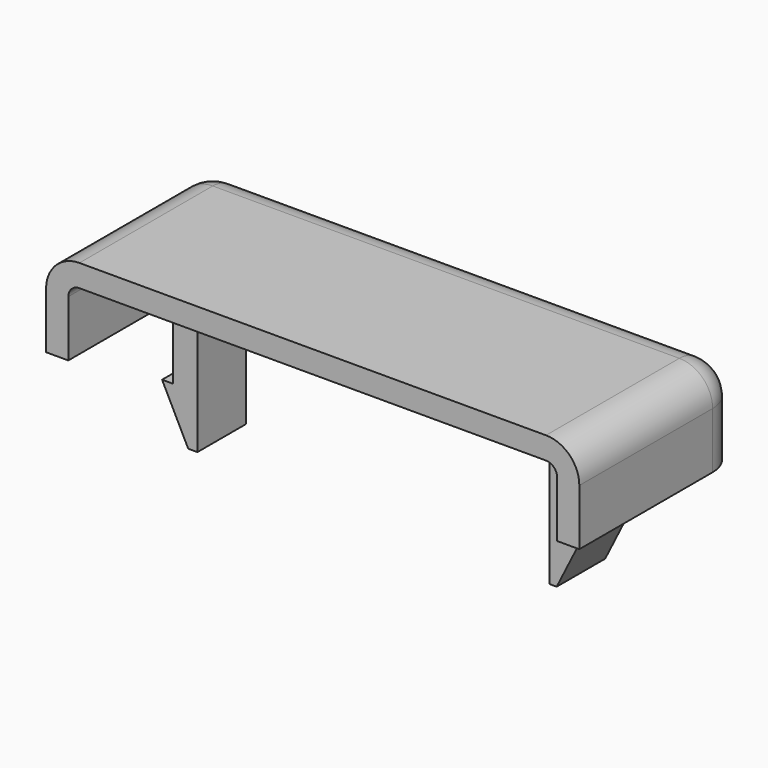
from build123d import *

# Parameters (mm, degrees)
F0_W         = 48
F0_H         = 8.0539090559
F1_DEPTH     = 18
F2_R         = 3
F3_T         = -2
F4_W         = 3.6368723959
F4_H         = 5.4553076625
F5_DEPTH     = 8
F6_W         = 3.8294224069
F6_H         = 5.4512945935
F7_DEPTH     = 8
F8_W         = 2.2997260094
F8_H         = 6.8176840032
F9_DEPTH     = 13.4
F8_W_2       = 2.9408568516
F11_T1_DEPTH = 36.529241079
F12_T1_DEPTH = 36.5332541479
F13_T1_DEPTH = 5.4512945935
F13_T3_DEPTH = 5.4553076625
F14_SIZE     = 1


# Not quite as in the source:
# - a fillet or chamfer that OpenCascade refuses, or shapes differently, is made with other operations: its cross-section is extruded or revolved along the edge and cut away or added


with BuildPart() as f1:
    # F0 (on Front) → F1 (new body)
    with BuildSketch(Plane.XZ):
        with Locations((7.3680209219, 4.0269545279)):
            Rectangle(F0_W, F0_H)
    extrude(amount=-F1_DEPTH)

    # F2
    f2_edges = [f1.edges().sort_by_distance(p)[0] for p in [
        (7.368021, 18, 8.053909),
        (-16.631979, 9, 8.053909),
        (31.368021, 9, 8.053909),
        (-16.631979, 18, 4.026955),
        (31.368021, 18, 4.026955),
    ]]
    fillet(f2_edges, radius=F2_R)

    # F3
    f3_openings = [f1.faces().sort_by_distance(p)[0] for p in [
        (7.368021, 0, 3.993074),
        (7.368021, 8.962591, 0),
    ]]
    offset(amount=F3_T, openings=f3_openings)

    # F4 (on Top) → F5 (join, symmetric)
    with BuildSketch(Plane.XY):
        with Locations((25.2722883597, 9.2779155821)):
            Rectangle(F4_W, F4_H)
    extrude(amount=F5_DEPTH, both=True)

    # F6 (on Top) → F7 (join, symmetric)
    with BuildSketch(Plane.XY):
        with Locations((-10.3424843401, 9.4998679124)):
            Rectangle(F6_W, F6_H)
    extrude(amount=F7_DEPTH, both=True)


with BuildPart() as f9:
    # F8 (on Front) → F9 (new body)
    with BuildSketch(Plane.XZ):
        with Locations((26.7013879493, 0.1128966487)):
            Rectangle(F8_W, F8_H)
    extrude(amount=-F9_DEPTH)


with BuildPart() as f9b:
    # F8 (on Front) → F9, piece 2 (new body)
    with BuildSketch(Plane.XZ):
        with Locations((-12.0930257253, 0.1128966487)):
            Rectangle(F8_W_2, F8_H)
    extrude(amount=-F9_DEPTH)


with BuildPart() as f1_1:
    add(f1.part)

    # F10: cut F9, F9b
    add(f9.part, mode=Mode.SUBTRACT)
    add(f9b.part, mode=Mode.SUBTRACT)

    # F11: chamfer of 6 x 3 on 1 edges, made by hand

    # F11_s2 → F11_t1 (cut)
    with BuildSketch(Plane.XZ.offset(-27.7644884519)):
        Polygon((-12.2571955435, -2), (-9.2571955435, -8), (-12.2571955435, -8), align=None)
    extrude(amount=F11_T1_DEPTH, mode=Mode.SUBTRACT)

    # F12: chamfer of 3 x 6 on 1 edges, made by hand

    # F12_s2 → F12_t1 (cut)
    with BuildSketch(Plane.XZ.offset(-27.544542656)):
        Polygon((27.0907245576, -2), (24.0907245576, -8), (27.0907245576, -8), align=None)
    extrude(amount=F12_T1_DEPTH, mode=Mode.SUBTRACT)

    # F13: fillet of radius 2 on 4 edges, made by hand

    # F13_s2 → F13_t1 (join)
    with BuildSketch(Plane.XZ.offset(-12.2255152091)):
        with BuildLine():
            ThreePointArc((-6.4277731366, 6.0539090559), (-7.841986699, 5.4681226183), (-8.4277731366, 4.0539090559))
            Line((-8.4277731366, 4.0539090559), (-8.4677731366, 4.0539090559))
            Line((-8.4677731366, 4.0539090559), (-8.4677731366, 6.0939090559))
            Line((-8.4677731366, 6.0939090559), (-6.4277731366, 6.0939090559))
            Line((-6.4277731366, 6.0939090559), (-6.4277731366, 6.0539090559))
        make_face()
        with BuildLine():
            ThreePointArc((-14.2571955435, 6.0539090559), (-12.8429819811, 5.4681226183), (-12.2571955435, 4.0539090559))
            Line((-12.2571955435, 4.0539090559), (-12.2171955435, 4.0539090559))
            Line((-12.2171955435, 4.0539090559), (-12.2171955435, 6.0939090559))
            Line((-12.2171955435, 6.0939090559), (-14.2571955435, 6.0939090559))
            Line((-14.2571955435, 6.0939090559), (-14.2571955435, 6.0539090559))
        make_face()
    extrude(amount=F13_T1_DEPTH)

    # F13_s4 → F13_t3 (join)
    with BuildSketch(Plane.XZ.offset(-12.0055694133)):
        with BuildLine():
            ThreePointArc((21.4538521618, 6.0539090559), (22.8680657241, 5.4681226183), (23.4538521618, 4.0539090559))
            Line((23.4538521618, 4.0539090559), (23.4938521618, 4.0539090559))
            Line((23.4938521618, 4.0539090559), (23.4938521618, 6.0939090559))
            Line((23.4938521618, 6.0939090559), (21.4538521618, 6.0939090559))
            Line((21.4538521618, 6.0939090559), (21.4538521618, 6.0539090559))
        make_face()
        with BuildLine():
            ThreePointArc((29.0907245576, 6.0539090559), (27.6765109953, 5.4681226183), (27.0907245576, 4.0539090559))
            Line((27.0907245576, 4.0539090559), (27.0507245576, 4.0539090559))
            Line((27.0507245576, 4.0539090559), (27.0507245576, 6.0939090559))
            Line((27.0507245576, 6.0939090559), (29.0907245576, 6.0939090559))
            Line((29.0907245576, 6.0939090559), (29.0907245576, 6.0539090559))
        make_face()
    extrude(amount=F13_T3_DEPTH)

    # F14
    f14_edges = [f1_1.edges().sort_by_distance(p)[0] for p in [
        (25.551525, 9.277916, 3.521739),
        (-10.622597, 9.499868, 3.521739),
    ]]
    chamfer(f14_edges, length=F14_SIZE)


solid = f1_1.part
